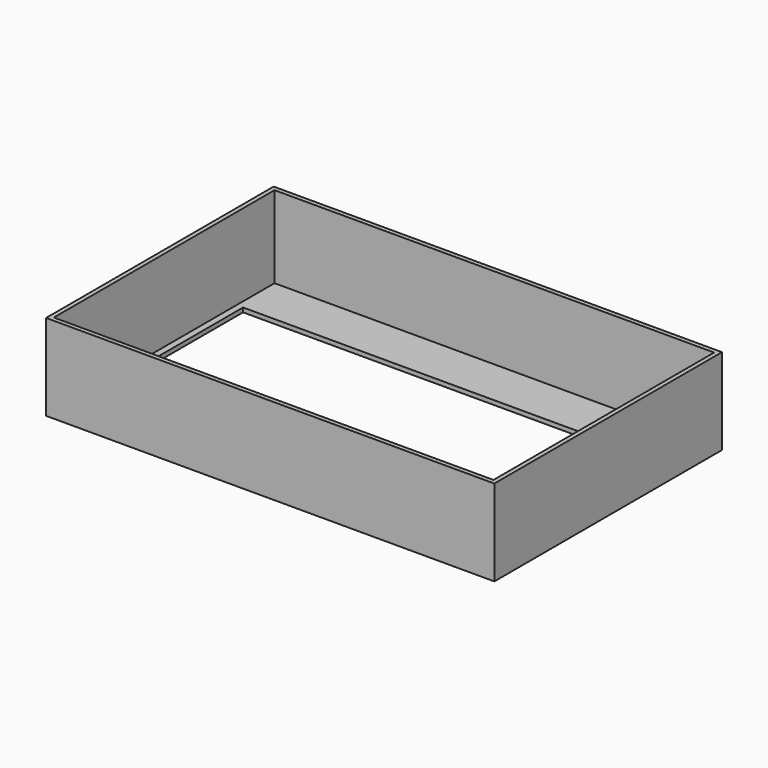
from build123d import *

# Parameters (mm, degrees)
F3_W     = 104
F3_H     = 66
F3_W_2   = 102
F3_H_2   = 64
F4_DEPTH = 20
F1_W     = 102
F1_H     = 64
F1_W_2   = 98.9999980927
F1_H_2   = 41.9999980927
F5_DEPTH = 1


# Not quite as in the source:
# - the program builds the solid bodies; features that only make, move or delete a surface that nothing else refers to are left out


with BuildPart() as f4:
    # F3 (on face) → F4 (new body)
    with BuildSketch(Plane.XY):
        with Locations((49, 30)):
            Rectangle(F3_W, F3_H)
        with Locations((49, 30)):
            Rectangle(F3_W_2, F3_H_2, mode=Mode.SUBTRACT)
    extrude(amount=F4_DEPTH)

    # F1 (on Top) → F5 (join)
    with BuildSketch(Plane.XY):
        with Locations((49, 30)):
            Rectangle(F1_W, F1_H)
        with Locations((49, 30)):
            Rectangle(F1_W_2, F1_H_2, mode=Mode.SUBTRACT)
    extrude(amount=F5_DEPTH)


solid = f4.part
